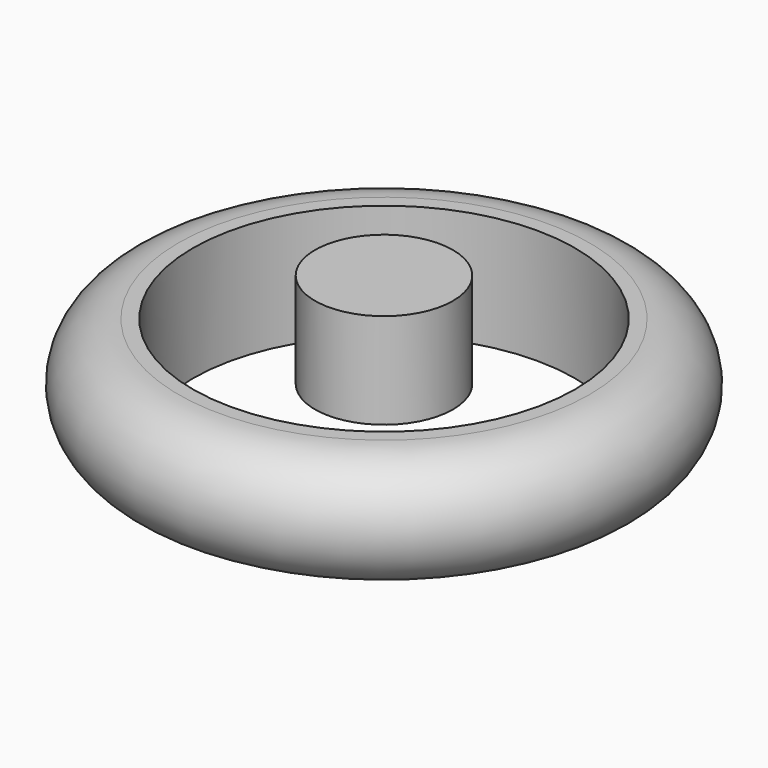
from build123d import *

# Parameters (mm, degrees)
F3_R     = 14.4288800287
F4_DEPTH = 20


# Not quite as in the source:
# - the program builds the solid bodies; features that only make, move or delete a surface that nothing else refers to are left out


with BuildPart() as f2:
    # F2: sweep along a path in F0
    with BuildLine(Plane.XY) as f2_path:
        CenterArc((0, 0), 40, 0, 360)
    # F1 (on Front) → F2 (sweep)
    with BuildSketch(Plane.XZ):
        with BuildLine():
            Line((-40, 12.0271782488), (-43, 12.0271782488))
            ThreePointArc((-43, 12.0271782488), (-55.2470707288, 0), (-43, -12.0271782488))
            Line((-43, -12.0271782488), (-40, -11.9728217512))
            Line((-40, -11.9728217512), (-40, 12.0271782488))
        make_face()
    sweep(path=f2_path.line)


with BuildPart() as f4:
    # F3 (on Top) → F4 (new body)
    with BuildSketch(Plane.XY):
        Circle(F3_R)
    extrude(amount=F4_DEPTH)


solid = Compound([f2.part, f4.part])
